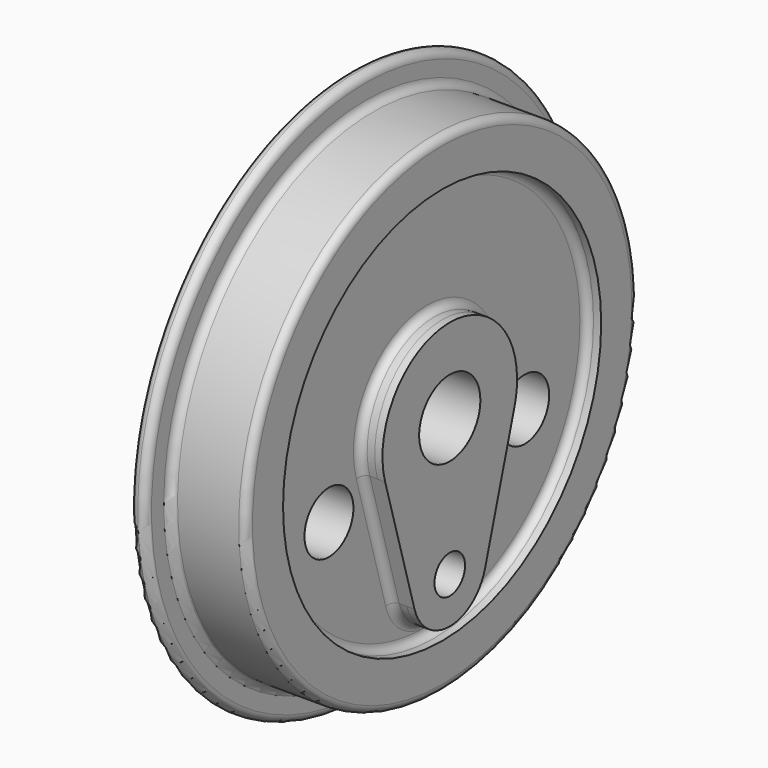
from build123d import *
from build123d import SkipClean  # not in build123d's __all__

# Parameters (mm, degrees)
F2_R     = 3.96875
F2_R_2   = 1.984375
F3_DEPTH = 0.79375
F4_R     = 1.984375
F5_DEPTH = 25.4
F6_R     = 3.175
F7_DEPTH = 25.4
F8_R     = 20.6375
F8_R_2   = 3.175
F9_DEPTH = 1.5875
F10_R    = 0.79374


# Not quite as in the source:
# - a fillet or chamfer is up to 0.001 mm smaller than in the source, because OpenCascade refuses the exact size


with BuildPart() as f1:
    # F0 (on Front) → F1 (revolve)
    with BuildSketch(Plane.XZ):
        with BuildLine():
            Line((20.1211371932, 32.3471946239), (10.5961371932, 32.3471946239))
            Line((10.5961371932, 32.3471946239), (10.5961371932, 8.5346946239))
            ThreePointArc((10.5961371932, 8.5346946239), (10.8286211857, 7.9734286164), (11.3898871932, 7.7409446239))
            ThreePointArc((11.3898871932, 7.7409446239), (11.9511532008, 7.9734286164), (12.1836371932, 8.5346946239))
            Line((12.1836371932, 8.5346946239), (12.1836371932, 10.1221946239))
            ThreePointArc((12.1836371932, 10.1221946239), (12.4161211857, 10.6834606315), (12.9773871932, 10.9159446239))
            Line((12.9773871932, 10.9159446239), (19.3273871932, 10.9159446239))
            ThreePointArc((19.3273871932, 10.9159446239), (19.8886532008, 11.1484286164), (20.1211371932, 11.7096946239))
            Line((20.1211371932, 11.7096946239), (20.1211371932, 32.3471946239))
        make_face()
    revolve(axis=Axis((22.0401428428, 0, 36.3159446239), (1, 0, 0)))

    # F2 (on face) → F3 (join)
    with BuildSketch(Plane.YZ.offset(20.1211371932)):
        with BuildLine():
            ThreePointArc((8.3876347926, 33.8905974017), (8.6449193994, 35.0911609125), (8.73125, 36.3159446239))
            ThreePointArc((8.73125, 36.3159446239), (-1.2247837114, 44.9608640234), (-8.3876347926, 33.8905974017))
            ThreePointArc((-8.3876347926, 33.8905974017), (0, 27.5846946239), (8.3876347926, 33.8905974017))
        make_face()
        with Locations((0, 36.3159446239)):
            Circle(F2_R, mode=Mode.SUBTRACT)
        with BuildLine():
            ThreePointArc((8.3876347926, 33.8905974017), (0, 27.5846946239), (-8.3876347926, 33.8905974017))
            Line((-8.3876347926, 33.8905974017), (-4.5750735232, 20.7055279573))
            ThreePointArc((-4.5750735232, 20.7055279573), (-0.6680638426, 26.7438552055), (4.7625, 22.0284446239))
            ThreePointArc((4.7625, 22.0284446239), (4.7154105815, 21.3603807814), (4.5750735232, 20.7055279573))
            Line((4.5750735232, 20.7055279573), (8.3876347926, 33.8905974017))
        make_face()
        with BuildLine():
            ThreePointArc((4.7625, 22.0284446239), (-0.6680638426, 26.7438552055), (-4.5750735232, 20.7055279573))
            ThreePointArc((-4.5750735232, 20.7055279573), (-2.8619063591, 18.221753378), (-8.55e-08, 17.2659446239))
            ThreePointArc((-8.55e-08, 17.2659446239), (2.8619062907, 18.2217533266), (4.5750735232, 20.7055279573))
            ThreePointArc((4.5750735232, 20.7055279573), (4.7154105815, 21.3603807814), (4.7625, 22.0284446239))
        make_face()
        with Locations((0, 22.0284446239)):
            Circle(F2_R_2, mode=Mode.SUBTRACT)
        with Locations((0, 22.0284446239)):
            Circle(F2_R_2)
    extrude(amount=F3_DEPTH)

    # F4 (on face) → F5 (cut)
    with BuildSketch(Plane.YZ.offset(20.9148871932)):
        with Locations((0, 22.0284446239)):
            Circle(F4_R)
    extrude(amount=-F5_DEPTH, mode=Mode.SUBTRACT)

    # F6 (on face) → F7 (cut)
    with BuildSketch(Plane.YZ.offset(20.1211371932)):
        with Locations((-12.7, 31.1710834503)):
            Circle(F6_R)
        with Locations((12.7, 31.1710834503)):
            Circle(F6_R)
    extrude(amount=-F7_DEPTH, mode=Mode.SUBTRACT)

    # F8 (on face) → F9 (cut)
    with BuildSketch(Plane.YZ.offset(20.1211371932)):
        with Locations((0, 36.3159446239)):
            Circle(F8_R)
        with Locations((-12.7, 31.1710834503)):
            Circle(F8_R_2, mode=Mode.SUBTRACT)
        with BuildLine():
            Line((-4.5750735232, 20.7055279573), (-8.3876347926, 33.8905974017))
            ThreePointArc((-8.3876347926, 33.8905974017), (0, 45.0471946239), (8.3876347926, 33.8905974017))
            Line((8.3876347926, 33.8905974017), (4.5750735232, 20.7055279573))
            ThreePointArc((4.5750735232, 20.7055279573), (0, 17.2659446239), (-4.5750735232, 20.7055279573))
        make_face(mode=Mode.SUBTRACT)
        with Locations((12.7, 31.1710834503)):
            Circle(F8_R_2, mode=Mode.SUBTRACT)
    with SkipClean():  # cleaning this boolean's faces spoils the solid; the shape is the same uncleaned
        extrude(amount=-F9_DEPTH, mode=Mode.SUBTRACT)

    # F10 (radius 0.79375 in the source; OpenCascade refuses exactly that, so slightly less here)
    f10_edges = [f1.edges().sort_by_distance(p)[0] for p in [
        (18.533637, -20.6375, 36.315945),
        (18.533637, 6.481354, 27.298063),
        (18.533637, 0, 45.047195),
        (18.533637, 0, 17.265945),
        (18.533637, -6.481354, 27.298063),
    ]]
    fillet(f10_edges, radius=F10_R)


solid = f1.part
